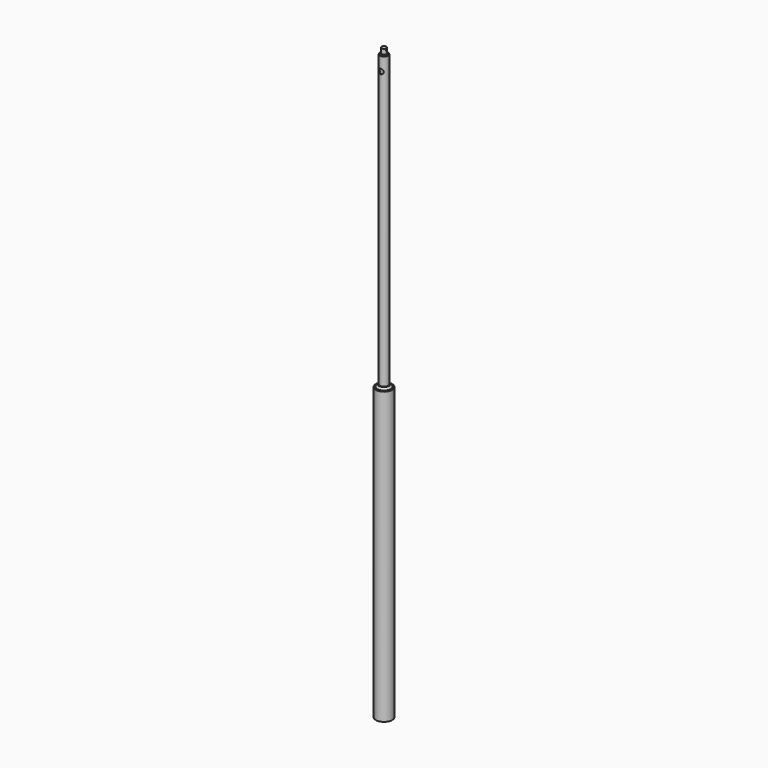
from build123d import *

# Parameters (mm, degrees)
F0_R      = 21
F0_R_2    = 17.5
F1_DEPTH  = 750
F2_R      = 17.5
F3_DEPTH  = 6
F4_R      = 10.65
F4_R_2    = 8.65
F5_DEPTH  = 750
F6_R      = 10.65
F6_R_2    = 8.65
F7_DEPTH  = 100
F9_R      = 17.5
F10_DEPTH = 6
F11_R     = 8.65
F12_DEPTH = 25
F13_R     = 6.35
F14_DEPTH = 15
F15_DEPTH = 15
F16_R     = 1.5
F17_DEPTH = 10
F18_R     = 8.65
F18_R_2   = 6.35
F19_DEPTH = 2
F20_R     = 6.35
F21_DEPTH = 21.001
F22_R     = 17.4
F22_R_2   = 10.75
F23_DEPTH = 100
F24_SIZE  = 5


with BuildPart() as f1:
    # F0 (on Top) → F1 (new body)
    with BuildSketch(Plane.XY):
        Circle(F0_R)
        Circle(F0_R_2, mode=Mode.SUBTRACT)
    extrude(amount=F1_DEPTH)

    # F9 (on offset) → F10 (join)
    with BuildSketch(Plane.XY.offset(650)):
        Circle(F9_R)
    extrude(amount=F10_DEPTH)


with BuildPart() as f3:
    # F2 (on face) → F3 (new body)
    with BuildSketch(Plane.XY.offset(750)):
        Circle(F2_R)
    extrude(amount=F3_DEPTH)

    # F24
    f24_edges = [f3.edges().sort_by_distance(p)[0] for p in [
        (-17.5, 0, 756),
    ]]
    chamfer(f24_edges, length=F24_SIZE)


with BuildPart() as f5:
    # F4 (on face) → F5 (new body)
    with BuildSketch(Plane.XY.offset(756)):
        Circle(F4_R)
        Circle(F4_R_2, mode=Mode.SUBTRACT)
    extrude(amount=F5_DEPTH)

    # F20 (on Front) → F21 (cut, through all)
    with BuildSketch(Plane.XZ):
        with Locations((0, 1471)):
            Circle(F20_R)
    extrude(amount=F21_DEPTH, mode=Mode.SUBTRACT)


with BuildPart() as f7:
    # F6 (on face) → F7 (new body)
    with BuildSketch(Plane.XY.offset(756)):
        Circle(F6_R)
        Circle(F6_R_2, mode=Mode.SUBTRACT)
    extrude(amount=-F7_DEPTH)


with BuildPart() as f12:
    # F11 (on face) → F12 (new body)
    with BuildSketch(Plane.XY.offset(1506)):
        Circle(F11_R)
    extrude(amount=-F12_DEPTH)

    # F13 (on face) → F14 (join)
    with BuildSketch(Plane.XY.offset(1506)):
        Circle(F13_R)
    extrude(amount=F14_DEPTH)

    # F13 (on face) → F15 (join)
    with BuildSketch(Plane.XY.offset(1506)):
        Circle(F13_R)
    extrude(amount=F15_DEPTH)

    # F16 (on Right) → F17 (cut, symmetric)
    with BuildSketch(Plane.YZ):
        with Locations((0, 1516.5)):
            Circle(F16_R)
    extrude(amount=F17_DEPTH, both=True, mode=Mode.SUBTRACT)

    # F18 (on face) → F19 (join)
    with BuildSketch(Plane.XY.offset(1506)):
        Circle(F18_R)
        Circle(F18_R_2, mode=Mode.SUBTRACT)
    extrude(amount=F19_DEPTH)


with BuildPart() as f23:
    # F22 (on face) → F23 (new body)
    with BuildSketch(Plane.XY.offset(750)):
        Circle(F22_R)
        Circle(F22_R_2, mode=Mode.SUBTRACT)
    extrude(amount=-F23_DEPTH)


solid = Compound([f1.part, f3.part, f5.part, f7.part, f12.part, f23.part])
